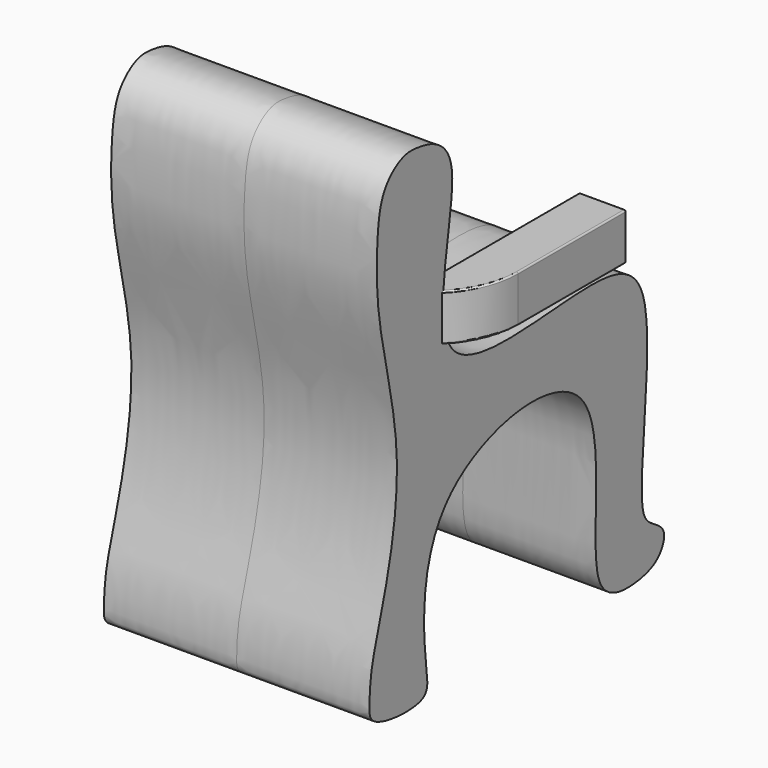
from build123d import *

# Parameters (mm, degrees)
F1_DEPTH     = 42.5
F3_W         = 15
F3_H         = 15
F7_T1_DEPTH  = 115.0662092469
F9_W         = 15
F9_H         = 15
F12_T1_DEPTH = 109.9375696185
F13_R        = 0.5
F14_R        = 0.5


# Not quite as in the source:
# - a fillet or chamfer that OpenCascade refuses, or shapes differently, is made with other operations: its cross-section is extruded or revolved along the edge and cut away or added


with BuildPart() as f1:
    # F0 (on Right) → F1 (new body, symmetric)
    with BuildSketch(Plane.YZ):
        with BuildLine():
            add(Edge.make_bspline(
                [(-40.0787331164, 10.499868542), (-49.57602414, 20.5272145255), (-35.215661923, 60.6016616211), (-46.1955440889, 72.1022070522), (-54.5329426018, 73.6348763119), (-60.4256466729, 73.9904615721), (-68.9380873459, 67.9088405183), (-71.0563389735, 53.6630140776), (-71.1235516335, 29.162139067), (-59.3350813457, -9.4337345876), (-67.0539239411, -46.6660335619), (-73.4151268835, -65.1291242845), (-73.868017569, -75.9133885238), (-73.7512176996, -83.079645184), (-49.4921585891, -85.2083420926), (-51.4253569792, -73.0646440198), (-56.1408447001, -20.5497802354), (30.4039784881, -6.6424695326), (8.7413251836, -84.0608343203), (33.1778175375, -85.3778788425), (42.6495555042, -81.9314615815), (45.3314729505, -74.170943153), (39.3579314396, -70.6611066554), (32.0121327758, -65.7037052209), (41.631739813, -10.9871619874), (26.6958326603, 14.4774590696), (-29.415487297, -0.7585055432), (-40.0787331164, 10.499868542)],
                knots=[0, 0, 0, 0, 0.062073, 0.0942145357, 0.118688218, 0.1396392145, 0.1662129636, 0.1985598187, 0.2420690717, 0.2984800238, 0.3528495859, 0.3916489453, 0.4197102692, 0.440305459, 0.4787895326, 0.5044921654, 0.5637072159, 0.6283664027, 0.6939933581, 0.7288144164, 0.7566621868, 0.778610157, 0.799604993, 0.8229397393, 0.8868545172, 0.9303064783, 1, 1, 1, 1], degree=3))
        make_face()
    extrude(amount=F1_DEPTH, both=True)

    # F6: sweep along a path in F5
    with BuildLine(Plane.YZ.offset(42.2)) as f6_path:
        Line((-44.71879825, 21.2678927928), (18.5077786446, 21.2678927928))
    # F3 (on offset) → F6 (sweep)
    with BuildSketch(Plane.XZ.offset(44.7)):
        with Locations((43.4150953591, 21.5689238906)):
            Rectangle(F3_W, F3_H)
    sweep(path=f6_path.line)

    # F7: fillet of radius 28.0048773235 on 1 edges, made by hand

    # F7_s2 → F7_t1 (cut)
    with BuildSketch(Plane.XY.offset(-35.9641807328)):
        with BuildLine():
            ThreePointArc((42.5002798094, -44.7190840938), (48.7261143137, -35.5609369059), (50.9154953591, -24.7055564046))
            Line((50.9154953591, -24.7055564046), (53.71611966, -24.7055564046))
            ThreePointArc((53.71611966, -24.7055564046), (53.71571966, -34.7121773273), (53.71571966, -44.71879825))
            Line((53.71571966, -44.71879825), (50.9150953591, -47.5194225509))
            ThreePointArc((50.9150953591, -47.5194225509), (46.7076875843, -47.5194225509), (44.4593825554, -46.7204368627))
            Line((44.4593825554, -46.7204368627), (42.5002798094, -44.7190840938))
        make_face()
    extrude(amount=F7_T1_DEPTH, mode=Mode.SUBTRACT)

    # F11: sweep along a path in F10
    with BuildLine(Plane.YZ.offset(-42.2)) as f11_path:
        Line((18.3076951653, 21.4679762721), (-45.5191358924, 21.4679762721))
    # F9 (on offset) → F11 (sweep)
    with BuildSketch(Plane.XZ.offset(44.7)):
        with Locations((-42.4209798872, 19.9641917646)):
            Rectangle(F9_W, F9_H)
    sweep(path=f11_path.line)

    # F12: fillet of radius 28.0005 on 1 edges, made by hand

    # F12_s2 → F12_t1 (cut)
    with BuildSketch(Plane.XY.offset(-35.0045930447)):
        with BuildLine():
            ThreePointArc((-42.5002939916, -45.5194071284), (-48.0002035451, -36.7248611659), (-49.9213798872, -26.5316219729))
            Line((-49.9213798872, -26.5316219729), (-52.7215664558, -26.5316219729))
            ThreePointArc((-52.7215664558, -26.5316219729), (-52.7211664558, -36.0253789326), (-52.7211664558, -45.5191358924))
            Line((-52.7211664558, -45.5191358924), (-49.9209798872, -48.3193224609))
            ThreePointArc((-49.9209798872, -48.3193224609), (-46.2106369394, -48.3193224609), (-44.5583719705, -47.4181856439))
            Line((-44.5583719705, -47.4181856439), (-42.5002939916, -45.5194071284))
        make_face()
    extrude(amount=F12_T1_DEPTH, mode=Mode.SUBTRACT)

    # F13
    f13_edges = [f1.edges().sort_by_distance(p)[0] for p in [
        (-49.92098, -4.186799, 27.464192),
        (-34.92098, -12.985998, 27.464192),
        (-42.42098, 18.307695, 12.464192),
        (-49.92098, -4.186799, 12.464192),
        (-49.92098, 18.307695, 19.964192),
        (-34.92098, 18.307695, 19.964192),
        (-42.42098, 18.307695, 27.464192),
        (-34.92098, -11.637629, 12.464192),
    ]]
    fillet(f13_edges, radius=F13_R)

    # F14
    f14_edges = [f1.edges().sort_by_distance(p)[0] for p in [
        (50.915095, -3.17373, 14.068924),
        (35.915095, -11.962876, 14.068924),
        (43.415095, 18.507779, 14.068924),
        (43.415095, 18.507779, 29.068924),
        (50.915095, 18.507779, 21.568924),
        (35.915095, 18.507779, 21.568924),
        (35.915095, -12.843402, 29.068924),
        (50.915095, -3.17373, 29.068924),
        (48.697093, -35.629701, 29.068924),
        (48.697093, -35.629701, 14.068924),
    ]]
    fillet(f14_edges, radius=F14_R)


solid = f1.part
